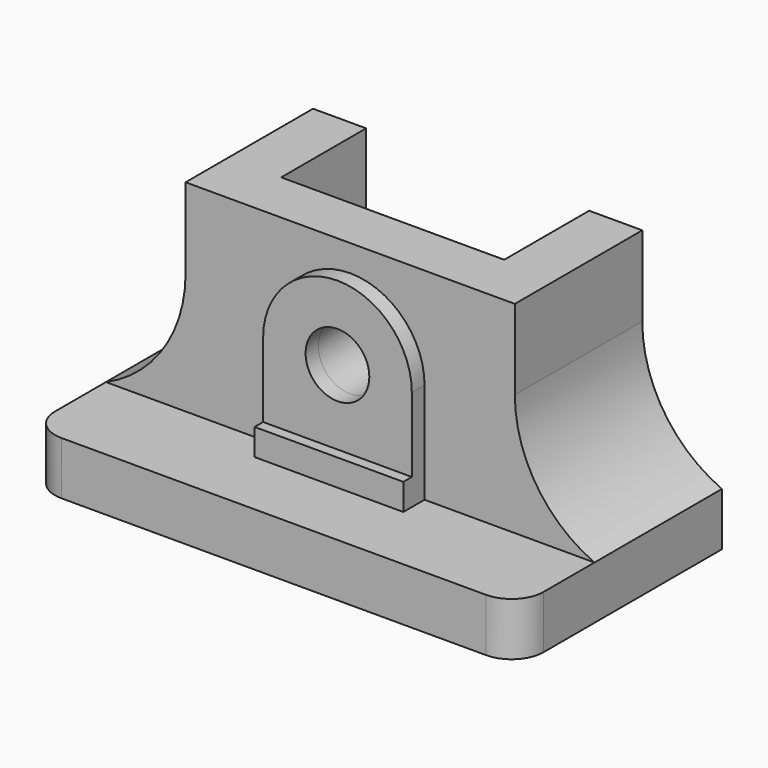
from build123d import *

# Parameters (mm, degrees)
F1_DEPTH    = 48
F2_DEPTH    = 10
F3_R        = 6
F4_T1_DEPTH = 30
F5_W        = 28
F5_H        = 5
F6_DEPTH    = 5
F5_R        = 6
F7_DEPTH    = 3
F8_DEPTH    = 30.001


# Not quite as in the source:
# - a fillet or chamfer that OpenCascade refuses, or shapes differently, is made with other operations: its cross-section is extruded or revolved along the edge and cut away or added


with BuildPart() as f1:
    # F0 (on Top) → F1 (new body)
    with BuildSketch(Plane.XY):
        Polygon((31, -6), (31, 24), (21, 24), (21, 4), (-21, 4), (-21, 24), (-31, 24), (-31, -6), align=None)
    extrude(amount=F1_DEPTH)

    # F0 (on Top) → F2 (join)
    with BuildSketch(Plane.XY):
        Polygon((-46, -24), (46, -24), (46, 24), (31, 24), (31, -6), (-31, -6), (-31, 24), (-46, 24), align=None)
        Polygon((31, -6), (31, 24), (21, 24), (21, 4), (-21, 4), (-21, 24), (-31, 24), (-31, -6), align=None)
    extrude(amount=F2_DEPTH)

    # F3
    f3_edges = [f1.edges().sort_by_distance(p)[0] for p in [
        (-46, -24, 5),
        (46, -24, 5),
    ]]
    fillet(f3_edges, radius=F3_R)

    # F4: fillet of radius 25 on 2 edges, made by hand

    # F4_s2 → F4_t1 (join)
    with BuildSketch(Plane.XZ.offset(-24)):
        with BuildLine():
            ThreePointArc((-46, 10), (-35.0834993366, 19.2198145372), (-31, 32.9128784748))
            Line((-31, 32.9128784748), (-31, 10))
            Line((-31, 10), (-46, 10))
        make_face()
        with BuildLine():
            ThreePointArc((46, 10), (35.0834993366, 19.2198145372), (31, 32.9128784748))
            Line((31, 32.9128784748), (31, 10))
            Line((31, 10), (46, 10))
        make_face()
    extrude(amount=F4_T1_DEPTH)

    # F5 (on face) → F6 (join)
    with BuildSketch(Plane.XZ.offset(6)):
        with Locations((0, 12.5)):
            Rectangle(F5_W, F5_H)
    extrude(amount=F6_DEPTH)

    # F5 (on face) → F7 (join)
    with BuildSketch(Plane.XZ.offset(6)):
        with BuildLine():
            Line((14, 15), (14, 29))
            ThreePointArc((14, 29), (0, 43), (-14, 29))
            Line((-14, 29), (-14, 15))
            Line((-14, 15), (14, 15))
        make_face()
        with Locations((0, 29)):
            Circle(F5_R, mode=Mode.SUBTRACT)
    extrude(amount=F7_DEPTH)

    # F8 (cut, through all): a face of the model
    f8_faces = [f1.faces().sort_by_distance(p)[0] for p in [
        (0, -6, 29),
    ]]
    extrude(f8_faces, amount=-F8_DEPTH, mode=Mode.SUBTRACT)


solid = f1.part
